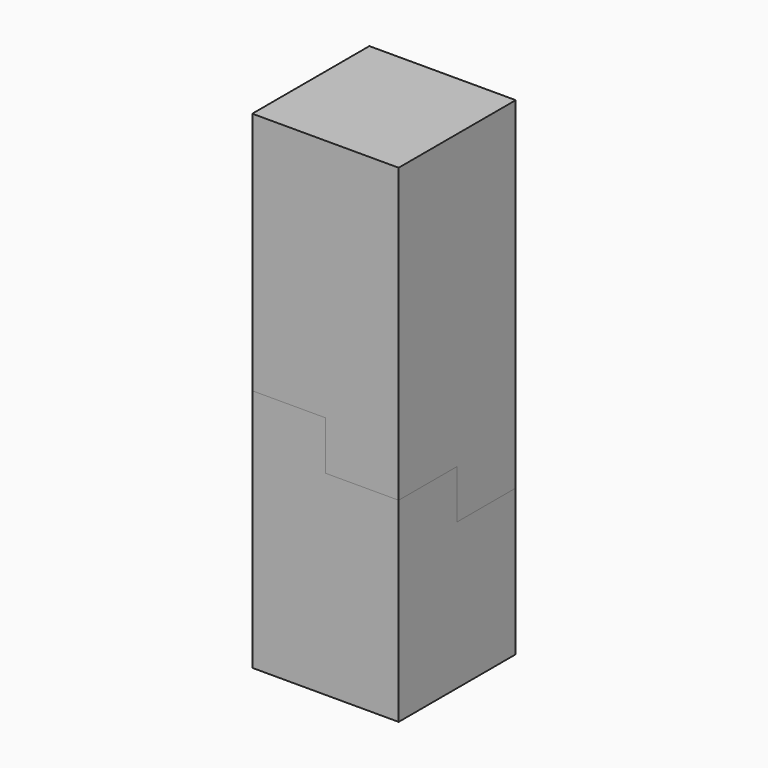
from build123d import *

# Parameters (mm, degrees)
F1_DEPTH  = 25.4
F2_DEPTH  = 38.1
F3_DEPTH  = 50.8
F4_DEPTH  = 63.5
F5_DEPTH  = 101.6
F7_DEPTH  = 101.6
F8_DEPTH  = 25.4
F9_DEPTH  = 38.1
F10_DEPTH = 50.8
F11_DEPTH = 63.5
F12_DEPTH = 76.2


with BuildPart() as f1:
    # F0 (on Top) → F1 (new body)
    with BuildSketch(Plane.XY):
        with BuildLine():
            Line((0, 38.1), (0, 19.05))
            Line((0, 19.05), (4.6619887504, 19.05))
            ThreePointArc((4.6619887504, 19.05), (8.8761396776, 29.2238603224), (19.05, 33.4380112496))
            Line((19.05, 33.4380112496), (19.05, 38.1))
            Line((19.05, 38.1), (0, 38.1))
        make_face()
    extrude(amount=F1_DEPTH)

    # F0 (on Top) → F2 (join)
    with BuildSketch(Plane.XY):
        with BuildLine():
            Line((33.4380112496, 19.05), (38.1, 19.05))
            Line((38.1, 19.05), (38.1, 38.1))
            Line((38.1, 38.1), (19.05, 38.1))
            Line((19.05, 38.1), (19.05, 33.4380112496))
            ThreePointArc((19.05, 33.4380112496), (29.2238603224, 29.2238603224), (33.4380112496, 19.05))
        make_face()
    extrude(amount=F2_DEPTH)

    # F0 (on Top) → F3 (join)
    with BuildSketch(Plane.XY):
        with BuildLine():
            Line((19.05, 4.6619887504), (19.05, 0))
            Line((19.05, 0), (38.1, 0))
            Line((38.1, 0), (38.1, 19.05))
            Line((38.1, 19.05), (33.4380112496, 19.05))
            ThreePointArc((33.4380112496, 19.05), (29.2238603224, 8.8761396776), (19.05, 4.6619887504))
        make_face()
    extrude(amount=F3_DEPTH)

    # F0 (on Top) → F4 (join)
    with BuildSketch(Plane.XY):
        with BuildLine():
            Line((0, 19.05), (0, 0))
            Line((0, 0), (19.05, 0))
            Line((19.05, 0), (19.05, 4.6619887504))
            ThreePointArc((19.05, 4.6619887504), (8.8761396776, 8.8761396776), (4.6619887504, 19.05))
            Line((4.6619887504, 19.05), (0, 19.05))
        make_face()
    extrude(amount=F4_DEPTH)

    # F0 (on Top) → F5 (join)
    with BuildSketch(Plane.XY):
        with BuildLine():
            ThreePointArc((19.05, 33.4380112496), (8.8761396776, 29.2238603224), (4.6619887504, 19.05))
            Line((4.6619887504, 19.05), (10.9808641353, 19.05))
            ThreePointArc((10.9808641353, 19.05), (13.3442593118, 24.7557406882), (19.05, 27.1191358647))
            Line((19.05, 27.1191358647), (19.05, 33.4380112496))
        make_face()
        with BuildLine():
            Line((27.1191358647, 19.05), (33.4380112496, 19.05))
            ThreePointArc((33.4380112496, 19.05), (29.2238603224, 29.2238603224), (19.05, 33.4380112496))
            Line((19.05, 33.4380112496), (19.05, 27.1191358647))
            ThreePointArc((19.05, 27.1191358647), (24.7557406882, 24.7557406882), (27.1191358647, 19.05))
        make_face()
        with BuildLine():
            Line((19.05, 10.9808641353), (19.05, 4.6619887504))
            ThreePointArc((19.05, 4.6619887504), (29.2238603224, 8.8761396776), (33.4380112496, 19.05))
            Line((33.4380112496, 19.05), (27.1191358647, 19.05))
            ThreePointArc((27.1191358647, 19.05), (24.7557406882, 13.3442593118), (19.05, 10.9808641353))
        make_face()
        with BuildLine():
            ThreePointArc((4.6619887504, 19.05), (8.8761396776, 8.8761396776), (19.05, 4.6619887504))
            Line((19.05, 4.6619887504), (19.05, 10.9808641353))
            ThreePointArc((19.05, 10.9808641353), (13.3442593118, 13.3442593118), (10.9808641353, 19.05))
            Line((10.9808641353, 19.05), (4.6619887504, 19.05))
        make_face()
    extrude(amount=F5_DEPTH)


with BuildPart() as f7:
    # F6 (on face) → F7 (new body, through all)
    with BuildSketch(Plane.XY.offset(101.6)):
        with BuildLine():
            Line((19.05, 19.05), (19.05, 26.3571361959))
            ThreePointArc((19.05, 26.3571361959), (13.8830744448, 24.2169255552), (11.7428638041, 19.05))
            Line((11.7428638041, 19.05), (19.05, 19.05))
        make_face()
        with BuildLine():
            Line((19.05, 19.05), (26.3571361959, 19.05))
            ThreePointArc((26.3571361959, 19.05), (24.2169255552, 24.2169255552), (19.05, 26.3571361959))
            Line((19.05, 26.3571361959), (19.05, 19.05))
        make_face()
        with BuildLine():
            ThreePointArc((11.7428638041, 19.05), (13.8830744448, 13.8830744448), (19.05, 11.7428638041))
            Line((19.05, 11.7428638041), (19.05, 19.05))
            Line((19.05, 19.05), (11.7428638041, 19.05))
        make_face()
        with BuildLine():
            ThreePointArc((19.05, 11.7428638041), (24.2169255552, 13.8830744448), (26.3571361959, 19.05))
            Line((26.3571361959, 19.05), (19.05, 19.05))
            Line((19.05, 19.05), (19.05, 11.7428638041))
        make_face()
    extrude(amount=-F7_DEPTH)

    # F6 (on face) → F8 (join)
    with BuildSketch(Plane.XY.offset(101.6)):
        with BuildLine():
            Line((38.1, 19.05), (33.4380112496, 19.05))
            ThreePointArc((33.4380112496, 19.05), (29.2238603224, 8.8761396776), (19.05, 4.6619887504))
            Line((19.05, 4.6619887504), (19.05, 0))
            Line((19.05, 0), (38.1, 0))
            Line((38.1, 0), (38.1, 19.05))
        make_face()
        with BuildLine():
            ThreePointArc((19.05, 4.6619887504), (29.2238603224, 8.8761396776), (33.4380112496, 19.05))
            Line((33.4380112496, 19.05), (27.1191358647, 19.05))
            ThreePointArc((27.1191358647, 19.05), (24.7557406882, 13.3442593118), (19.05, 10.9808641353))
            Line((19.05, 10.9808641353), (19.05, 4.6619887504))
        make_face()
        with BuildLine():
            ThreePointArc((19.05, 10.9808641353), (24.7557406882, 13.3442593118), (27.1191358647, 19.05))
            Line((27.1191358647, 19.05), (26.3571361959, 19.05))
            ThreePointArc((26.3571361959, 19.05), (24.2169255552, 13.8830744448), (19.05, 11.7428638041))
            Line((19.05, 11.7428638041), (19.05, 10.9808641353))
        make_face()
        with BuildLine():
            ThreePointArc((19.05, 11.7428638041), (24.2169255552, 13.8830744448), (26.3571361959, 19.05))
            Line((26.3571361959, 19.05), (19.05, 19.05))
            Line((19.05, 19.05), (19.05, 11.7428638041))
        make_face()
        with BuildLine():
            ThreePointArc((11.7428638041, 19.05), (13.8830744448, 13.8830744448), (19.05, 11.7428638041))
            Line((19.05, 11.7428638041), (19.05, 19.05))
            Line((19.05, 19.05), (11.7428638041, 19.05))
        make_face()
        with BuildLine():
            ThreePointArc((10.9808641353, 19.05), (13.3442593118, 13.3442593118), (19.05, 10.9808641353))
            Line((19.05, 10.9808641353), (19.05, 11.7428638041))
            ThreePointArc((19.05, 11.7428638041), (13.8830744448, 13.8830744448), (11.7428638041, 19.05))
            Line((11.7428638041, 19.05), (10.9808641353, 19.05))
        make_face()
        with BuildLine():
            ThreePointArc((4.6619887504, 19.05), (8.8761396776, 8.8761396776), (19.05, 4.6619887504))
            Line((19.05, 4.6619887504), (19.05, 10.9808641353))
            ThreePointArc((19.05, 10.9808641353), (13.3442593118, 13.3442593118), (10.9808641353, 19.05))
            Line((10.9808641353, 19.05), (4.6619887504, 19.05))
        make_face()
        with BuildLine():
            Line((19.05, 0), (19.05, 4.6619887504))
            ThreePointArc((19.05, 4.6619887504), (8.8761396776, 8.8761396776), (4.6619887504, 19.05))
            Line((4.6619887504, 19.05), (0, 19.05))
            Line((0, 19.05), (0, 0))
            Line((0, 0), (19.05, 0))
        make_face()
        with BuildLine():
            Line((19.05, 19.05), (19.05, 26.3571361959))
            ThreePointArc((19.05, 26.3571361959), (13.8830744448, 24.2169255552), (11.7428638041, 19.05))
            Line((11.7428638041, 19.05), (19.05, 19.05))
        make_face()
        with BuildLine():
            Line((19.05, 26.3571361959), (19.05, 27.1191358647))
            ThreePointArc((19.05, 27.1191358647), (13.3442593118, 24.7557406882), (10.9808641353, 19.05))
            Line((10.9808641353, 19.05), (11.7428638041, 19.05))
            ThreePointArc((11.7428638041, 19.05), (13.8830744448, 24.2169255552), (19.05, 26.3571361959))
        make_face()
        with BuildLine():
            Line((19.05, 27.1191358647), (19.05, 33.4380112496))
            ThreePointArc((19.05, 33.4380112496), (8.8761396776, 29.2238603224), (4.6619887504, 19.05))
            Line((4.6619887504, 19.05), (10.9808641353, 19.05))
            ThreePointArc((10.9808641353, 19.05), (13.3442593118, 24.7557406882), (19.05, 27.1191358647))
        make_face()
        with BuildLine():
            ThreePointArc((4.6619887504, 19.05), (8.8761396776, 29.2238603224), (19.05, 33.4380112496))
            Line((19.05, 33.4380112496), (19.05, 38.1))
            Line((19.05, 38.1), (0, 38.1))
            Line((0, 38.1), (0, 19.05))
            Line((0, 19.05), (4.6619887504, 19.05))
        make_face()
        with BuildLine():
            Line((19.05, 19.05), (26.3571361959, 19.05))
            ThreePointArc((26.3571361959, 19.05), (24.2169255552, 24.2169255552), (19.05, 26.3571361959))
            Line((19.05, 26.3571361959), (19.05, 19.05))
        make_face()
        with BuildLine():
            Line((26.3571361959, 19.05), (27.1191358647, 19.05))
            ThreePointArc((27.1191358647, 19.05), (24.7557406882, 24.7557406882), (19.05, 27.1191358647))
            Line((19.05, 27.1191358647), (19.05, 26.3571361959))
            ThreePointArc((19.05, 26.3571361959), (24.2169255552, 24.2169255552), (26.3571361959, 19.05))
        make_face()
        with BuildLine():
            Line((27.1191358647, 19.05), (33.4380112496, 19.05))
            ThreePointArc((33.4380112496, 19.05), (29.2238603224, 29.2238603224), (19.05, 33.4380112496))
            Line((19.05, 33.4380112496), (19.05, 27.1191358647))
            ThreePointArc((19.05, 27.1191358647), (24.7557406882, 24.7557406882), (27.1191358647, 19.05))
        make_face()
        with BuildLine():
            ThreePointArc((19.05, 33.4380112496), (29.2238603224, 29.2238603224), (33.4380112496, 19.05))
            Line((33.4380112496, 19.05), (38.1, 19.05))
            Line((38.1, 19.05), (38.1, 38.1))
            Line((38.1, 38.1), (19.05, 38.1))
            Line((19.05, 38.1), (19.05, 33.4380112496))
        make_face()
    extrude(amount=F8_DEPTH)

    # F6 (on face) → F9 (join, through all)
    with BuildSketch(Plane.XY.offset(101.6)):
        with BuildLine():
            Line((19.05, 0), (19.05, 4.6619887504))
            ThreePointArc((19.05, 4.6619887504), (8.8761396776, 8.8761396776), (4.6619887504, 19.05))
            Line((4.6619887504, 19.05), (0, 19.05))
            Line((0, 19.05), (0, 0))
            Line((0, 0), (19.05, 0))
        make_face()
    extrude(amount=-F9_DEPTH)

    # F6 (on face) → F10 (join, through all)
    with BuildSketch(Plane.XY.offset(101.6)):
        with BuildLine():
            Line((38.1, 19.05), (33.4380112496, 19.05))
            ThreePointArc((33.4380112496, 19.05), (29.2238603224, 8.8761396776), (19.05, 4.6619887504))
            Line((19.05, 4.6619887504), (19.05, 0))
            Line((19.05, 0), (38.1, 0))
            Line((38.1, 0), (38.1, 19.05))
        make_face()
    extrude(amount=-F10_DEPTH)

    # F6 (on face) → F11 (join, through all)
    with BuildSketch(Plane.XY.offset(101.6)):
        with BuildLine():
            ThreePointArc((19.05, 33.4380112496), (29.2238603224, 29.2238603224), (33.4380112496, 19.05))
            Line((33.4380112496, 19.05), (38.1, 19.05))
            Line((38.1, 19.05), (38.1, 38.1))
            Line((38.1, 38.1), (19.05, 38.1))
            Line((19.05, 38.1), (19.05, 33.4380112496))
        make_face()
    extrude(amount=-F11_DEPTH)

    # F6 (on face) → F12 (join, through all)
    with BuildSketch(Plane.XY.offset(101.6)):
        with BuildLine():
            ThreePointArc((4.6619887504, 19.05), (8.8761396776, 29.2238603224), (19.05, 33.4380112496))
            Line((19.05, 33.4380112496), (19.05, 38.1))
            Line((19.05, 38.1), (0, 38.1))
            Line((0, 38.1), (0, 19.05))
            Line((0, 19.05), (4.6619887504, 19.05))
        make_face()
    extrude(amount=-F12_DEPTH)


solid = Compound([f1.part, f7.part])
